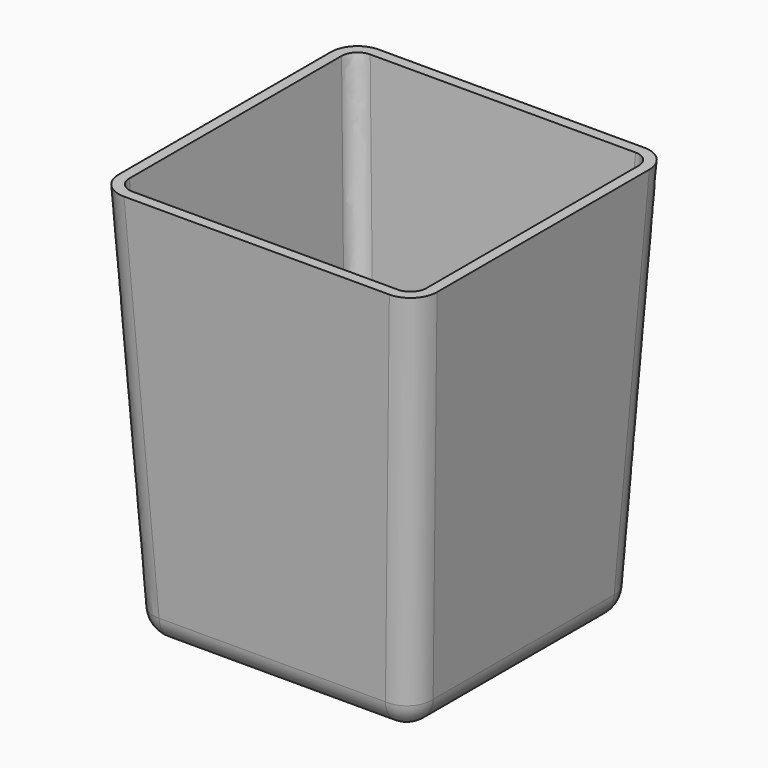
from build123d import *

# Parameters (mm, degrees)
F0_W     = 60
F0_H     = 60
F1_DEPTH = 75
F1_TAPER = 3
F2_R     = 5
F3_T     = 2
F5_DEPTH = 10
F6_R     = 2
F7_D     = 3.3
F7_DEPTH = 30.0010001
F8_D     = 3.3


# Not quite as in the source:
# - a shell that OpenCascade refuses in one call is made with other operations: the cavity is built on its own and cut out


with BuildPart() as f1:
    # F0 (on Top) → F1 (new body)
    with BuildSketch(Plane.XY):
        Rectangle(F0_W, F0_H)
    extrude(amount=-F1_DEPTH, taper=F1_TAPER)

    # F2
    f2_edges = [f1.edges().sort_by_distance(p)[0] for p in [
        (28.034708, 28.034708, -37.5),
        (-28.034708, 28.034708, -37.5),
        (-28.034708, -28.034708, -37.5),
        (28.034708, -28.034708, -37.5),
        (26.069417, 0, -75),
        (0, 26.069417, -75),
        (-26.069417, 0, -75),
        (0, -26.069417, -75),
    ]]
    fillet(f2_edges, radius=F2_R)

    # F3: shell of thickness 2, made by hand


with BuildPart() as f3_core1:
    # F3_t2: copy of F1
    add(f1.part)

    # the walls: a layer under each face that stays
    f3_faces = [f3_core1.faces().sort_by_distance(p)[0] for p in [
        (28.158870697, 0, -35.1308398906),
        (26.6944131636, -26.6944131636, -35.1847826561),
        (26.6944131636, 26.6944131636, -35.1847826561),
        (24.7663665987, 0, -73.6268718551),
        (0, -28.158870697, -35.1308398906),
        (0, 28.158870697, -35.1308398906),
        (-26.6944131636, -26.6944131636, -35.1847826561),
        (-26.6944131636, 26.6944131636, -35.1847826561),
        (-28.158870697, 0, -35.1308398906),
        (23.7582946672, -23.7582949577, -73.626871653),
        (23.7582946672, 23.7582949577, -73.626871653),
        (0, 0, -75),
        (0, -24.7663665987, -73.6268718551),
        (0, 24.7663665987, -73.6268718551),
        (-23.7582946672, -23.7582949577, -73.626871653),
        (-23.7582949577, 23.7582946672, -73.626871653),
        (-24.7663665987, 0, -73.6268718551),
    ]]
    thicken(f3_faces, amount=-F3_T, mode=Mode.SUBTRACT)


with BuildPart() as f1_1:
    add(f1.part)

    # what is left inside the walls is the cavity
    f3_cavity = [f3_core1.part.solids().sort_by_distance(p)[0] for p in [
        (0, 26.751692, -23.384623),
    ]]
    add(f3_cavity, mode=Mode.SUBTRACT)

    # F4 (on Right) → F5 (join, symmetric)
    with BuildSketch(Plane.YZ):
        Polygon((5, -83), (13, -75), (-13, -75), (-5, -83), align=None)
    extrude(amount=F5_DEPTH, both=True)

    # F6
    f6_edges = [f1_1.edges().sort_by_distance(p)[0] for p in [
        (-10, -9, -79),
        (-10, 0, -83),
        (-10, 9, -79),
        (10, 9, -79),
        (10, 0, -83),
        (10, -9, -79),
        (0, -5, -83),
        (0, 5, -83),
    ]]
    fillet(f6_edges, radius=F6_R)

    # F7 (through all, one way)
    with BuildSketch(Plane.YZ):
        with Locations((0, -78)):
            Circle(F7_D / 2)
    extrude(amount=-F7_DEPTH, mode=Mode.SUBTRACT)

    # F8 (through all)
    with Locations(Plane(origin=(0, 0, 0), x_dir=(0, 1, 0), z_dir=(-1, 0, 0))):
        with Locations((0, 78)):
            Hole(F8_D / 2)


solid = f1_1.part
